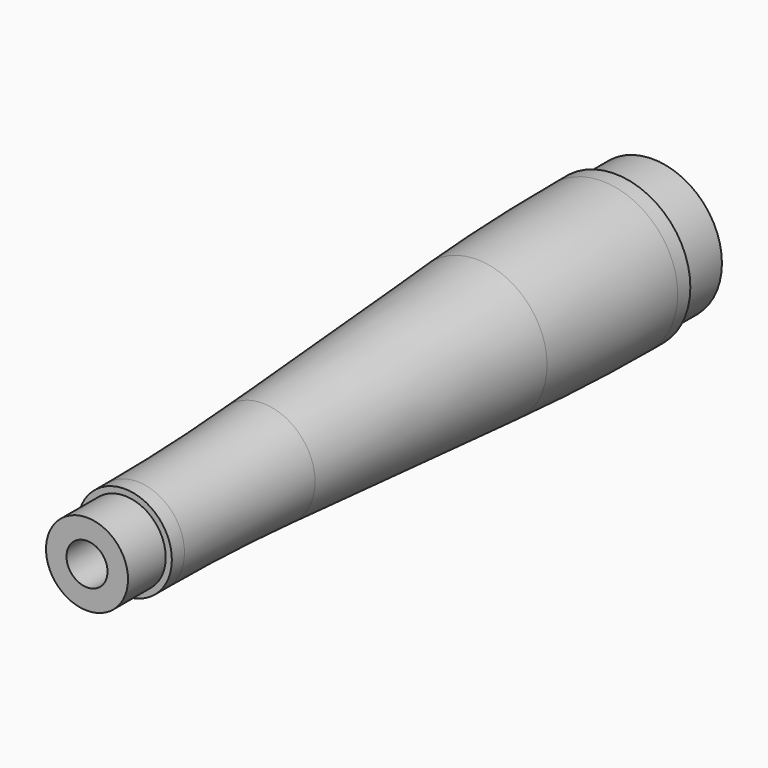
from build123d import *


# Not quite as in the source:
# - a fillet or chamfer that OpenCascade refuses, or shapes differently, is made with other operations: its cross-section is extruded or revolved along the edge and cut away or added


with BuildPart() as f1:
    # F0 (on Top) → F1 (revolve)
    with BuildSketch(Plane.XY):
        Polygon((14.7, 0), (4.35, 0), (4.35, -12), (9.35, -17), (6.35, -136), (4.35, -138), (4.35, -150), (8.7, -150), (8.7, -140), (10, -140), (10, -120), (16, -30), (16, -10), (14.7, -10), align=None)
    revolve(axis=Axis((0, -75, 0), (0, 1, 0)))

    # F2: fillet of radius 500 on 2 edges, made by hand

    # F2_s1 → F2_t2 (revolve, cut)
    with BuildSketch(Plane.XY):
        with BuildLine():
            ThreePointArc((14.8925789283, -46.6113160754), (15.7230680408, -29.9907791687), (16, -13.3518108135))
            Line((16, -13.3518108135), (16, -30))
            Line((16, -30), (14.8925789283, -46.6113160754))
        make_face()
    revolve(axis=Axis((0, -30, 0), (0, 1, 0)), mode=Mode.SUBTRACT)

    # F2_s3 → F2_t4 (revolve)
    with BuildSketch(Plane.XY):
        with BuildLine():
            ThreePointArc((11.1074210717, -103.3886839246), (10.2769319592, -120.0092208313), (10, -136.6481891865))
            Line((10, -136.6481891865), (10, -120))
            Line((10, -120), (11.1074210717, -103.3886839246))
        make_face()
    revolve(axis=Axis((0, -120, 0), (0, 1, 0)))


solid = f1.part
